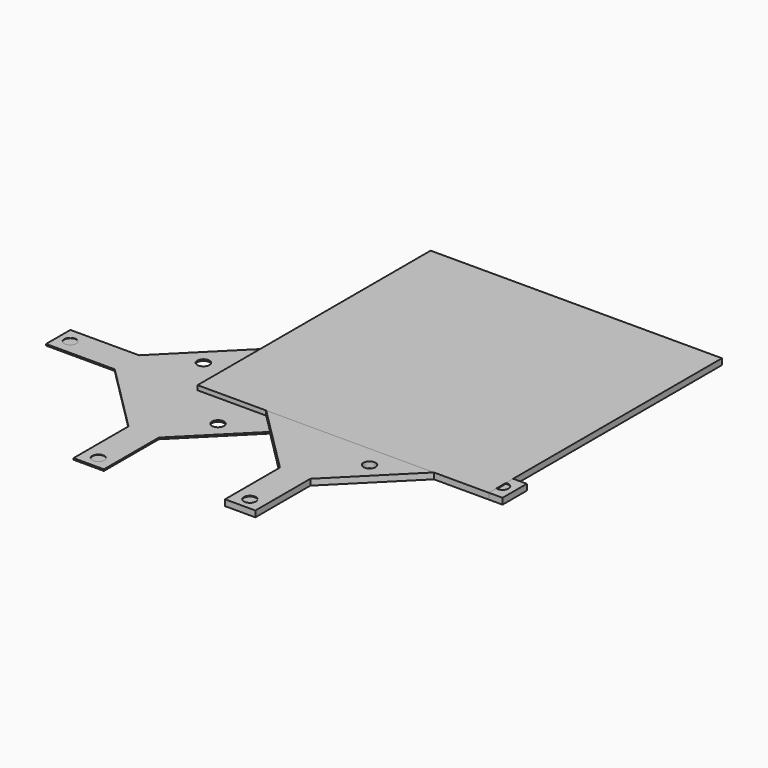
from build123d import *

# Parameters (mm, degrees)
F0_W      = 304.8
F0_H      = 304.8
F1_DEPTH  = 6.35
F3_DEPTH  = 6.35
F4_R      = 6.35
F5_DEPTH  = 25.4
F6_R      = 6.35
F7_DEPTH  = 0.79375
F9_DEPTH  = 1.5875
F10_R     = 6.35
F11_DEPTH = 25.4
F12_R     = 6.35
F13_DEPTH = 0.396875
F14_W     = 304.8
F14_H     = 304.8
F15_DEPTH = 6.35


with BuildPart() as f1:
    # F0 (on Top) → F1 (new body)
    with BuildSketch(Plane.XY):
        with Locations((152.4, 152.4)):
            Rectangle(F0_W, F0_H)
    extrude(amount=F1_DEPTH)


with BuildPart() as f3:
    # F2 (on Top) → F3 (new body)
    with BuildSketch(Plane.XY):
        Polygon((0, 31.75), (0, 0), (71.8420489686, 0), (143.6840979371, -71.8420489686), (143.6840979371, -143.6840979371), (175.4340979371, -143.6840979371), (175.4340979371, -71.8420489686), (247.2761469057, 0), (319.1181958742, 0), (319.1181958742, 31.75), (247.2761469057, 31.75), (175.4340979371, 103.5920489686), (175.4340979371, 175.4340979371), (143.6840979371, 175.4340979371), (143.6840979371, 103.5920489686), (71.8420489686, 31.75), align=None)
    extrude(amount=F3_DEPTH)

    # F4 (on face) → F5 (cut)
    with BuildSketch(Plane.XY.offset(6.35)):
        with Locations((197.8826454177, -22.4527331247)):
            Circle(F4_R)
        with Locations((119.9405228485, 52.9077055167)):
            Circle(F4_R)
    extrude(amount=-F5_DEPTH, mode=Mode.SUBTRACT)

    # F6 (on face) → F7 (cut)
    with BuildSketch(Plane.XY.offset(6.35)):
        with Locations((12.7, 15.875)):
            Circle(F6_R)
        with Locations((159.5590979371, 162.7340979371)):
            Circle(F6_R)
        with Locations((306.4181958742, 15.875)):
            Circle(F6_R)
        with Locations((159.5590979371, -130.9840979371)):
            Circle(F6_R)
    extrude(amount=-F7_DEPTH, mode=Mode.SUBTRACT)


with BuildPart() as f9:
    # F8 (on Top) → F9 (new body)
    with BuildSketch(Plane.XY):
        Polygon((-147.9062711463, 18.5312063838), (-147.9062711463, -13.2187936162), (-76.0642221777, -13.2187936162), (-4.2221732092, -85.0608425847), (-4.2221732092, -156.9028915533), (27.5278267908, -156.9028915533), (27.5278267908, -85.0608425847), (99.3698757594, -13.2187936162), (171.2119247279, -13.2187936162), (171.2119247279, 18.5312063838), (99.3698757594, 18.5312063838), (27.5278267908, 90.3732553524), (27.5278267908, 162.2153043209), (-4.2221732092, 162.2153043209), (-4.2221732092, 90.3732553524), (-76.0642221777, 18.5312063838), align=None)
    extrude(amount=F9_DEPTH)

    # F10 (on face) → F11 (cut)
    with BuildSketch(Plane.XY.offset(1.5875)):
        with Locations((49.9763742715, -35.6715267409)):
            Circle(F10_R)
        with Locations((-26.6749063339, 40.9797538644)):
            Circle(F10_R)
    extrude(amount=-F11_DEPTH, mode=Mode.SUBTRACT)

    # F12 (on face) → F13 (cut)
    with BuildSketch(Plane.XY.offset(1.5875)):
        with Locations((11.6528267908, 149.5153043209)):
            Circle(F12_R)
        with Locations((-135.2062711463, 2.6562063838)):
            Circle(F12_R)
        with Locations((158.5119247279, 2.6562063838)):
            Circle(F12_R)
        with Locations((11.6528267908, -144.2028915533)):
            Circle(F12_R)
    extrude(amount=-F13_DEPTH, mode=Mode.SUBTRACT)


with BuildPart() as f15:
    # F14 (on Top) → F15 (new body)
    with BuildSketch(Plane.XY):
        with Locations((152.4, 152.4)):
            Rectangle(F14_W, F14_H)
    extrude(amount=F15_DEPTH)


solid = Compound([f1.part, f3.part, f9.part, f15.part])
